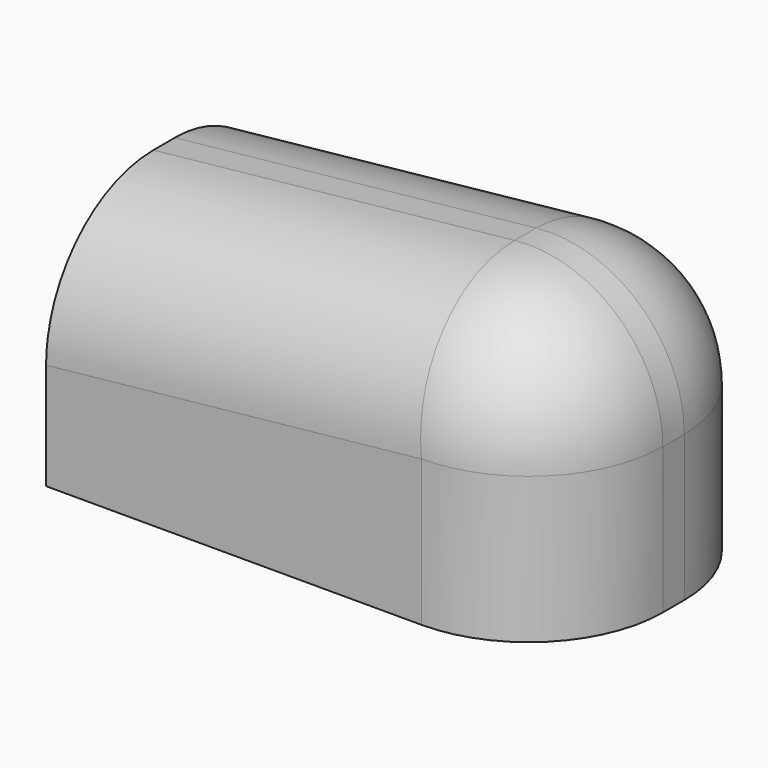
from build123d import *

# Parameters (mm, degrees)
F0_W     = 19
F0_H     = 11
F1_DEPTH = 11
F3_DEPTH = 25
F4_R     = 5


with BuildPart() as f1:
    # F0 (on Top) → F1 (new body)
    with BuildSketch(Plane.XY):
        Rectangle(F0_W, F0_H)
    extrude(amount=F1_DEPTH)

    # F2 (on face) → F3 (cut)
    with BuildSketch(Plane.XZ.offset(5.5)):
        Polygon((-9.5, 11), (-9.5, 9), (9.5, 11), align=None)
    extrude(amount=-F3_DEPTH, mode=Mode.SUBTRACT)

    # F4
    f4_edges = [f1.edges().sort_by_distance(p)[0] for p in [
        (0, -5.5, 10),
        (9.5, 0, 11),
        (0, 5.5, 10),
        (9.5, -5.5, 5.5),
        (9.5, 5.5, 5.5),
    ]]
    fillet(f4_edges, radius=F4_R)


solid = f1.part
